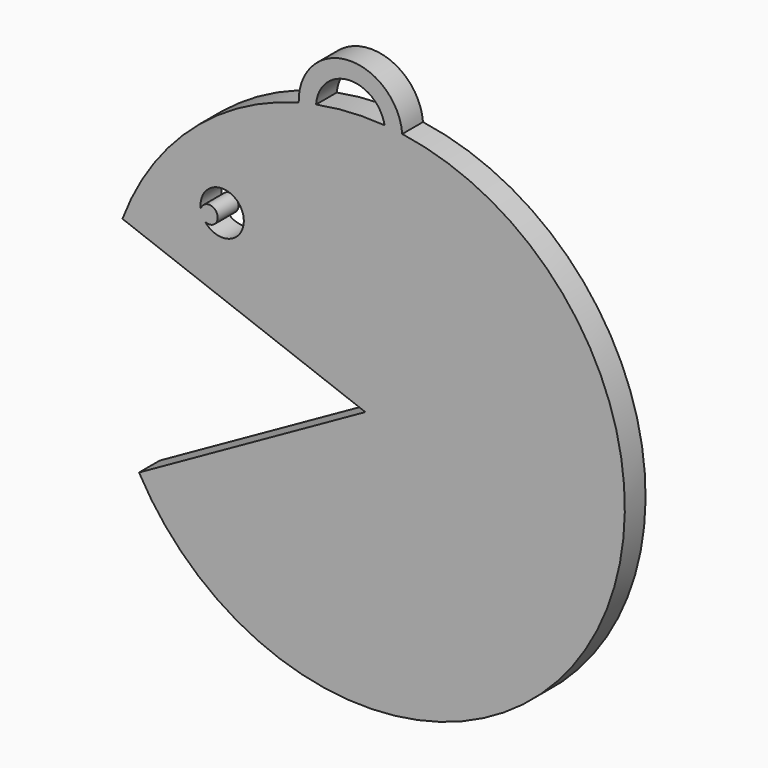
from build123d import *

# Parameters (mm, degrees)
F0_R         = 2.5
F1_DEPTH     = 3
F2_TEXT_SIZE = 11.1580619382
F3_DEPTH     = 1
F4_R         = 1
F5_DEPTH     = 3


# Not quite as in the source:
# - Text() gives the source's letters only with a copy of the font that has no kerning and outlines rounded to 1/6400 em; it was checked with that copy


with BuildPart() as f1:
    # F0 (on Front) → F1 (new body)
    with BuildSketch(Plane.XZ):
        with BuildLine():
            Line((43.6447212372, 30.0523352095), (17.4717715154, 15.3902513583))
            ThreePointArc((17.4717715154, 15.3902513583), (68.3805487788, 13.0776824639), (47.9113038938, 59.7473898893))
            ThreePointArc((47.9113038938, 59.7473898893), (46.8898802724, 59.8763011235), (45.8646348476, 59.9700888612))
            ThreePointArc((45.8646348476, 59.9700888612), (41.8884338593, 60.0008819964), (37.9430871765, 59.50554164))
            ThreePointArc((37.9430871765, 59.50554164), (36.9358317236, 59.2925609524), (35.9364772875, 59.0451442354))
            ThreePointArc((35.9364772875, 59.0451442354), (23.5075199978, 52.2895366126), (15.5561189336, 40.5894325627))
            Line((15.5561189336, 40.5894325627), (43.6447212372, 30.0523352095))
        make_face()
        with Locations((27.090748772, 44.9332743883)):
            Circle(F0_R, mode=Mode.SUBTRACT)
        with BuildLine():
            ThreePointArc((45.8646348476, 59.9700888612), (46.8898802724, 59.8763011235), (47.9113038938, 59.7473898893))
            ThreePointArc((47.9113038938, 59.7473898893), (41.58235806, 65.2201448079), (35.9364772875, 59.0451442354))
            ThreePointArc((35.9364772875, 59.0451442354), (36.9358317236, 59.2925609524), (37.9430871765, 59.50554164))
            ThreePointArc((37.9430871765, 59.50554164), (41.6994438852, 63.2235750221), (45.8646348476, 59.9700888612))
        make_face()
    extrude(amount=F1_DEPTH)

    # F2 (on face) → F3 (cut)
    with BuildSketch(Plane(origin=(0, 0, 0), x_dir=(-1, 0, 0), z_dir=(0, 1, 0))):
        with Locations((-62.5923797488, 9.4087719917)):
            Text('samuel', F2_TEXT_SIZE, font='Open Sans', text_align=(TextAlign.LEFT, TextAlign.BOTTOM))
    extrude(amount=-F3_DEPTH, mode=Mode.SUBTRACT)

    # F4 (on face) → F5 (join, through all)
    with BuildSketch(Plane.XZ.offset(3)):
        with Locations((25.5715490802, 44.2894325627)):
            Circle(F4_R)
    extrude(amount=-F5_DEPTH)


solid = f1.part
